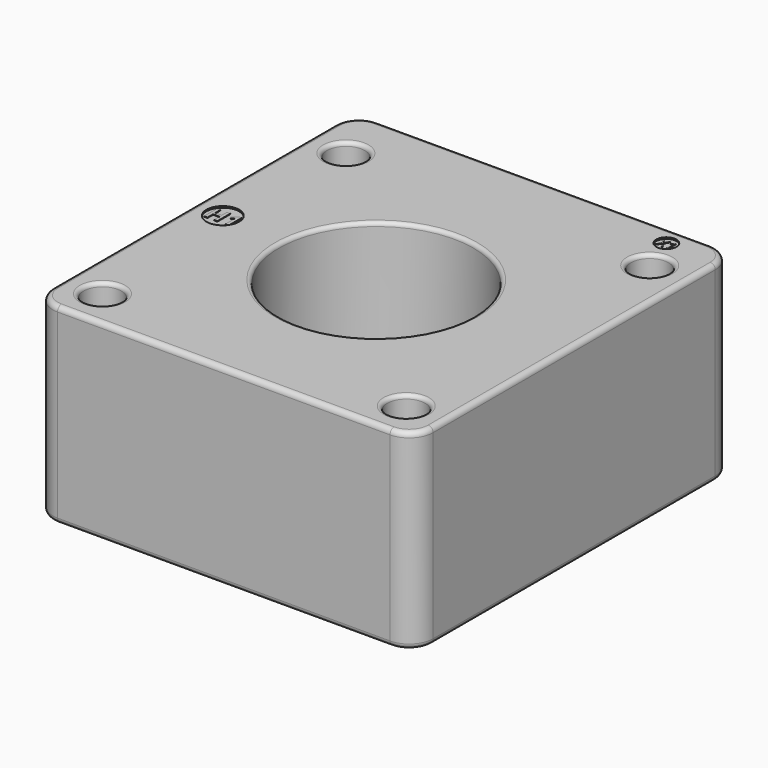
from build123d import *

# Parameters (mm, degrees)
F0_W          = 151
F0_H          = 159
F0_R          = 7.5
F0_R_2        = 38.625
F1_DEPTH      = 76
F2_W          = 9.5
F2_H          = 9.5
F3_DEPTH      = 1.5
F4_R          = 2.05
F5_R          = 2.05
F6_DEPTH      = 9.25
F7_R          = 6.5
F7_R_2        = 4
F8_DEPTH      = 0.6
F9_TEXT_SIZE  = 9.0491565629
F10_DEPTH     = 0.2
F11_TEXT_SIZE = 5.6605579125
F12_DEPTH     = 0.2
F13_R         = 2
F14_T1_DEPTH  = 76
F14_T4_ANGLE  = 90
F14_T6_ANGLE  = 90
F14_T8_ANGLE  = 90
F14_T10_ANGLE = 90
F14_T12_ANGLE = 90
F14_T14_ANGLE = 90
F14_T16_ANGLE = 90
F14_T18_ANGLE = 90
F15_R         = 1.5


# Not quite as in the source:
# - a fillet or chamfer that OpenCascade refuses, or shapes differently, is made with other operations: its cross-section is extruded or revolved along the edge and cut away or added
# - Text() gives the source's letters only with a copy of the font that has no kerning and outlines rounded to 1/6400 em; it was checked with that copy


with BuildPart() as f1:
    # F0 (on Top) → F1 (new body)
    with BuildSketch(Plane.XY):
        Rectangle(F0_W, F0_H)
        with Locations((-60.4, -64.2)):
            Circle(F0_R, mode=Mode.SUBTRACT)
        with Locations((60.2, -64.2)):
            Circle(F0_R, mode=Mode.SUBTRACT)
        with Locations((0, -3.875)):
            Circle(F0_R_2, mode=Mode.SUBTRACT)
        with Locations((-60.4, 56.6)):
            Circle(F0_R, mode=Mode.SUBTRACT)
        with Locations((60.2, 56.6)):
            Circle(F0_R, mode=Mode.SUBTRACT)
    extrude(amount=F1_DEPTH)

    # F2 (on face) → F3 (join)
    with BuildSketch(Plane(origin=(0, 79.5, 0), x_dir=(-1, 0, 0), z_dir=(0, 1, 0))):
        with Locations((-34.25, 38)):
            Rectangle(F2_W, F2_H)
        with Locations((-53.25, 38)):
            Rectangle(F2_W, F2_H)
    extrude(amount=F3_DEPTH)

    # F4 (on face) + F5 (on face) → F6 (join)
    with BuildSketch(Plane(origin=(0, 81, 0), x_dir=(-1, 0, 0), z_dir=(0, 1, 0))):
        with Locations((-34.25, 38)):
            Circle(F4_R)
    with BuildSketch(Plane(origin=(0, 81, 0), x_dir=(-1, 0, 0), z_dir=(0, 1, 0))):
        with Locations((-53.25, 38)):
            Circle(F5_R)
    extrude(amount=F6_DEPTH)

    # F7 (on face) → F8 (cut)
    with BuildSketch(Plane.XY.offset(76)):
        with Locations((-64, 0)):
            Circle(F7_R)
        with Locations((54.9, 71.5)):
            Circle(F7_R_2)
    extrude(amount=-F8_DEPTH, mode=Mode.SUBTRACT)

    # F9 (on face) → F10 (join)
    with BuildSketch(Plane.XY.offset(75.4)):
        with Locations((-69.6412769495, -3.2864618838)):
            Text('H1', F9_TEXT_SIZE, font='Open Sans', font_style=FontStyle.BOLD, text_align=(TextAlign.LEFT, TextAlign.BOTTOM))
    extrude(amount=F10_DEPTH)

    # F11 (on face) → F12 (join)
    with BuildSketch(Plane.XY.offset(75.4)):
        with Locations((51.7744719982, 69.5223361254)):
            Text('X1', F11_TEXT_SIZE, font='Open Sans', text_align=(TextAlign.LEFT, TextAlign.BOTTOM))
    extrude(amount=F12_DEPTH)

    # F13
    f13_edges = [f1.edges().sort_by_distance(p)[0] for p in [
        (0, 79.5, 76),
        (0, 79.5, 0),
        (75.5, 0, 76),
        (0, -79.5, 76),
        (-75.5, 0, 76),
        (75.5, 0, 0),
        (0, -79.5, 0),
        (-75.5, 0, 0),
    ]]
    fillet(f13_edges, radius=F13_R)

    # F14: fillet of radius 9.5 on 4 edges, made by hand

    # F14_s2 → F14_t1 (cut)
    with BuildSketch(Plane.XY):
        with BuildLine():
            ThreePointArc((75.5, 70), (72.7175144213, 76.7175144213), (66, 79.5))
            Line((66, 79.5), (75.5, 79.5))
            Line((75.5, 79.5), (75.5, 70))
        make_face()
        with BuildLine():
            ThreePointArc((-75.5, 70), (-72.7175144213, 76.7175144213), (-66, 79.5))
            Line((-66, 79.5), (-75.5, 79.5))
            Line((-75.5, 79.5), (-75.5, 70))
        make_face()
        with BuildLine():
            ThreePointArc((-66, -79.5), (-72.7175144213, -76.7175144213), (-75.5, -70))
            Line((-75.5, -70), (-75.5, -79.5))
            Line((-75.5, -79.5), (-66, -79.5))
        make_face()
        with BuildLine():
            ThreePointArc((66, -79.5), (72.7175144213, -76.7175144213), (75.5, -70))
            Line((75.5, -70), (75.5, -79.5))
            Line((75.5, -79.5), (66, -79.5))
        make_face()
    extrude(amount=F14_T1_DEPTH, mode=Mode.SUBTRACT)

    # F14_s3 → F14_t4 (revolve, cut)
    with BuildSketch(Plane.XZ.offset(70)):
        with BuildLine():
            ThreePointArc((73.5, 0), (74.9142135624, 0.5857864376), (75.5, 2))
            Line((75.5, 2), (75.5, 0))
            Line((75.5, 0), (73.5, 0))
        make_face()
    revolve(axis=Axis((66, -70, 0), (0, 0, -1)), revolution_arc=F14_T4_ANGLE, mode=Mode.SUBTRACT)

    # F14_s5 → F14_t6 (revolve, cut)
    with BuildSketch(Plane.YZ.offset(66)):
        with BuildLine():
            ThreePointArc((-77.5, 76), (-78.9142135624, 75.4142135624), (-79.5, 74))
            Line((-79.5, 74), (-79.5, 76))
            Line((-79.5, 76), (-77.5, 76))
        make_face()
    revolve(axis=Axis((66, -70, 76), (0, 0, 1)), revolution_arc=F14_T6_ANGLE, mode=Mode.SUBTRACT)

    # F14_s7 → F14_t8 (revolve, cut)
    with BuildSketch(Plane.YZ.offset(-66)):
        with BuildLine():
            ThreePointArc((-77.5, 0), (-78.9142135624, 0.5857864376), (-79.5, 2))
            Line((-79.5, 2), (-79.5, 0))
            Line((-79.5, 0), (-77.5, 0))
        make_face()
    revolve(axis=Axis((-66, -70, 0), (0, 0, -1)), revolution_arc=F14_T8_ANGLE, mode=Mode.SUBTRACT)

    # F14_s9 → F14_t10 (revolve, cut)
    with BuildSketch(Plane.XZ.offset(70)):
        with BuildLine():
            ThreePointArc((-73.5, 76), (-74.9142135624, 75.4142135624), (-75.5, 74))
            Line((-75.5, 74), (-75.5, 76))
            Line((-75.5, 76), (-73.5, 76))
        make_face()
    revolve(axis=Axis((-66, -70, 76), (0, 0, 1)), revolution_arc=F14_T10_ANGLE, mode=Mode.SUBTRACT)

    # F14_s11 → F14_t12 (revolve, cut)
    with BuildSketch(Plane.XZ.offset(-70)):
        with BuildLine():
            ThreePointArc((-73.5, 0), (-74.9142135624, 0.5857864376), (-75.5, 2))
            Line((-75.5, 2), (-75.5, 0))
            Line((-75.5, 0), (-73.5, 0))
        make_face()
    revolve(axis=Axis((-66, 70, 0), (0, 0, -1)), revolution_arc=F14_T12_ANGLE, mode=Mode.SUBTRACT)

    # F14_s13 → F14_t14 (revolve, cut)
    with BuildSketch(Plane.YZ.offset(-66)):
        with BuildLine():
            ThreePointArc((77.5, 76), (78.9142135624, 75.4142135624), (79.5, 74))
            Line((79.5, 74), (79.5, 76))
            Line((79.5, 76), (77.5, 76))
        make_face()
    revolve(axis=Axis((-66, 70, 76), (0, 0, 1)), revolution_arc=F14_T14_ANGLE, mode=Mode.SUBTRACT)

    # F14_s15 → F14_t16 (revolve, cut)
    with BuildSketch(Plane.YZ.offset(66)):
        with BuildLine():
            ThreePointArc((77.5, 0), (78.9142135624, 0.5857864376), (79.5, 2))
            Line((79.5, 2), (79.5, 0))
            Line((79.5, 0), (77.5, 0))
        make_face()
    revolve(axis=Axis((66, 70, 0), (0, 0, -1)), revolution_arc=F14_T16_ANGLE, mode=Mode.SUBTRACT)

    # F14_s17 → F14_t18 (revolve, cut)
    with BuildSketch(Plane.XZ.offset(-70)):
        with BuildLine():
            ThreePointArc((73.5, 76), (74.9142135624, 75.4142135624), (75.5, 74))
            Line((75.5, 74), (75.5, 76))
            Line((75.5, 76), (73.5, 76))
        make_face()
    revolve(axis=Axis((66, 70, 76), (0, 0, 1)), revolution_arc=F14_T18_ANGLE, mode=Mode.SUBTRACT)

    # F15
    f15_edges = [f1.edges().sort_by_distance(p)[0] for p in [
        (52.7, 56.6, 0),
        (52.7, -64.2, 0),
        (-38.625, -3.875, 0),
        (-67.9, -64.2, 0),
        (-67.9, 56.6, 0),
        (-38.625, -3.875, 76),
        (52.7, 56.6, 76),
        (-67.9, 56.6, 76),
        (-67.9, -64.2, 76),
        (52.7, -64.2, 76),
    ]]
    fillet(f15_edges, radius=F15_R)


solid = f1.part
